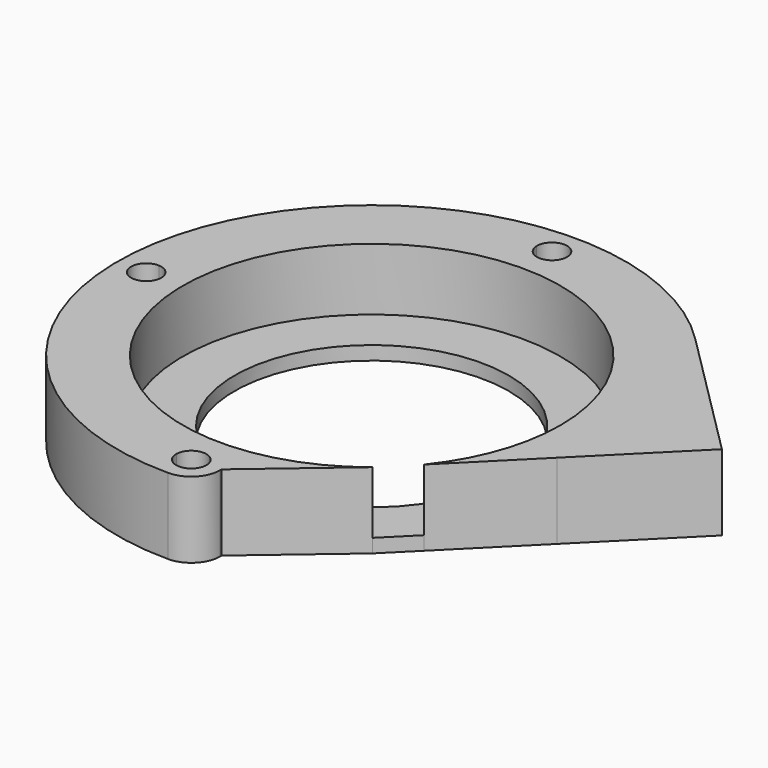
from build123d import *

# Parameters (mm, degrees)
F0_R     = 15
F1_DEPTH = 1.5
F2_DEPTH = 6.8


with BuildPart() as f1:
    # F0 (on Top) → F1 (new body)
    with BuildSketch(Plane.XY):
        with BuildLine():
            ThreePointArc((24.1652138662, -4.8646622494), (24.5285040494, -2.4443790825), (24.65, 0))
            ThreePointArc((24.65, 0), (18.0037803541, 16.8370541652), (1.6490756219, 24.5947768763))
            ThreePointArc((1.6490756219, 24.5947768763), (0, 23), (-1.6490756219, 24.5947768763))
            ThreePointArc((-1.6490756219, 24.5947768763), (-17.4301821562, 17.4301821562), (-24.5947768763, 1.6490756219))
            ThreePointArc((-24.5947768763, 1.6490756219), (-23.4639101733, 1.1470357113), (-23, 0))
            ThreePointArc((-23, 0), (-23.4639101733, -1.1470357113), (-24.5947768763, -1.6490756219))
            ThreePointArc((-24.5947768763, -1.6490756219), (-17.9529932576, -16.8911969112), (-3.1435634706, -24.4487322515))
            ThreePointArc((-3.1435634706, -24.4487322515), (0, -21.5), (3.1435634706, -24.4487322515))
            Line((3.1435634706, -24.4487322515), (12.969203616, -16.0692954907))
            ThreePointArc((12.969203616, -16.0692954907), (-18.6311104697, 8.9052918349), (20.65, 0))
            ThreePointArc((20.65, 0), (19.4738226895, -6.8696964896), (16.0792755585, -12.9568282197))
            Line((16.0792755585, -12.9568282197), (24.1652138662, -4.8646622494))
        make_face()
        with BuildLine():
            ThreePointArc((1.6490756219, 24.5947768763), (18.0037803541, 16.8370541652), (24.65, 0))
            ThreePointArc((24.65, 0), (24.5285040494, -2.4443790825), (24.1652138662, -4.8646622494))
            Line((24.1652138662, -4.8646622494), (27.771636901, -1.2554616043))
            ThreePointArc((27.771636901, -1.2554616043), (27.7929083207, -0.6278909749), (27.8, 0))
            ThreePointArc((27.8, 0), (25.6818028962, 10.6435426433), (19.65, 19.6651341211))
            ThreePointArc((19.65, 19.6651341211), (-25.6858981613, 10.6336557988), (7.1e-09, -27.8))
            ThreePointArc((7.1e-09, -27.8), (-2.2974435124, -26.8050529709), (-3.1435634706, -24.4487322515))
            ThreePointArc((-3.1435634706, -24.4487322515), (-17.9529932576, -16.8911969112), (-24.5947768763, -1.6490756219))
            ThreePointArc((-24.5947768763, -1.6490756219), (-26.3, 0), (-24.5947768763, 1.6490756219))
            ThreePointArc((-24.5947768763, 1.6490756219), (-17.4301821562, 17.4301821562), (-1.6490756219, 24.5947768763))
            ThreePointArc((-1.6490756219, 24.5947768763), (-0.0276154299, 26.2997688893), (1.65, 24.65))
            ThreePointArc((1.65, 24.65), (1.6497688893, 24.6223845701), (1.6490756219, 24.5947768763))
        make_face()
        with BuildLine():
            ThreePointArc((3.15, -24.65), (3.1483904564, -24.549314679), (3.1435634706, -24.4487322515))
            ThreePointArc((3.1435634706, -24.4487322515), (2.3974318813, -24.5331371898), (1.6490756219, -24.5947768763))
            ThreePointArc((1.6490756219, -24.5947768763), (1.6497688893, -24.6223845701), (1.65, -24.65))
            ThreePointArc((1.65, -24.65), (-0.0276154299, -26.2997688893), (-1.6490756219, -24.5947768763))
            ThreePointArc((-1.6490756219, -24.5947768763), (-2.3974318813, -24.5331371898), (-3.1435634706, -24.4487322515))
            ThreePointArc((-3.1435634706, -24.4487322515), (-2.2974435124, -26.8050529709), (7.1e-09, -27.8))
            ThreePointArc((7.1e-09, -27.8), (2.2273863633, -26.8773863582), (3.15, -24.65))
        make_face()
        with BuildLine():
            ThreePointArc((1.6490756219, -24.5947768763), (2.3974318813, -24.5331371898), (3.1435634706, -24.4487322515))
            ThreePointArc((3.1435634706, -24.4487322515), (0, -21.5), (-3.1435634706, -24.4487322515))
            ThreePointArc((-3.1435634706, -24.4487322515), (-2.3974318813, -24.5331371898), (-1.6490756219, -24.5947768763))
            ThreePointArc((-1.6490756219, -24.5947768763), (0, -23), (1.6490756219, -24.5947768763))
        make_face()
        with BuildLine():
            Line((12.969203616, -16.0692954907), (16.0792755585, -12.9568282197))
            ThreePointArc((16.0792755585, -12.9568282197), (19.4738226895, -6.8696964896), (20.65, 0))
            ThreePointArc((20.65, 0), (-18.6311104697, 8.9052918349), (12.969203616, -16.0692954907))
        make_face()
        Circle(F0_R, mode=Mode.SUBTRACT)
        with BuildLine():
            ThreePointArc((27.8, 0), (27.7929083207, -0.6278909749), (27.771636901, -1.2554616043))
            Line((27.771636901, -1.2554616043), (34.1742395873, 5.1520722659))
            Line((34.1742395873, 5.1520722659), (19.65, 19.6651341211))
            ThreePointArc((19.65, 19.6651341211), (25.6818028962, 10.6435426433), (27.8, 0))
        make_face()
    extrude(amount=-F1_DEPTH)

    # F0 (on Top) → F2 (join)
    with BuildSketch(Plane.XY):
        with BuildLine():
            ThreePointArc((24.1652138662, -4.8646622494), (24.5285040494, -2.4443790825), (24.65, 0))
            ThreePointArc((24.65, 0), (18.0037803541, 16.8370541652), (1.6490756219, 24.5947768763))
            ThreePointArc((1.6490756219, 24.5947768763), (0, 23), (-1.6490756219, 24.5947768763))
            ThreePointArc((-1.6490756219, 24.5947768763), (-17.4301821562, 17.4301821562), (-24.5947768763, 1.6490756219))
            ThreePointArc((-24.5947768763, 1.6490756219), (-23.4639101733, 1.1470357113), (-23, 0))
            ThreePointArc((-23, 0), (-23.4639101733, -1.1470357113), (-24.5947768763, -1.6490756219))
            ThreePointArc((-24.5947768763, -1.6490756219), (-17.9529932576, -16.8911969112), (-3.1435634706, -24.4487322515))
            ThreePointArc((-3.1435634706, -24.4487322515), (0, -21.5), (3.1435634706, -24.4487322515))
            Line((3.1435634706, -24.4487322515), (12.969203616, -16.0692954907))
            ThreePointArc((12.969203616, -16.0692954907), (-18.6311104697, 8.9052918349), (20.65, 0))
            ThreePointArc((20.65, 0), (19.4738226895, -6.8696964896), (16.0792755585, -12.9568282197))
            Line((16.0792755585, -12.9568282197), (24.1652138662, -4.8646622494))
        make_face()
        with BuildLine():
            ThreePointArc((1.6490756219, 24.5947768763), (18.0037803541, 16.8370541652), (24.65, 0))
            ThreePointArc((24.65, 0), (24.5285040494, -2.4443790825), (24.1652138662, -4.8646622494))
            Line((24.1652138662, -4.8646622494), (27.771636901, -1.2554616043))
            ThreePointArc((27.771636901, -1.2554616043), (27.7929083207, -0.6278909749), (27.8, 0))
            ThreePointArc((27.8, 0), (25.6818028962, 10.6435426433), (19.65, 19.6651341211))
            ThreePointArc((19.65, 19.6651341211), (-25.6858981613, 10.6336557988), (7.1e-09, -27.8))
            ThreePointArc((7.1e-09, -27.8), (-2.2974435124, -26.8050529709), (-3.1435634706, -24.4487322515))
            ThreePointArc((-3.1435634706, -24.4487322515), (-17.9529932576, -16.8911969112), (-24.5947768763, -1.6490756219))
            ThreePointArc((-24.5947768763, -1.6490756219), (-26.3, 0), (-24.5947768763, 1.6490756219))
            ThreePointArc((-24.5947768763, 1.6490756219), (-17.4301821562, 17.4301821562), (-1.6490756219, 24.5947768763))
            ThreePointArc((-1.6490756219, 24.5947768763), (-0.0276154299, 26.2997688893), (1.65, 24.65))
            ThreePointArc((1.65, 24.65), (1.6497688893, 24.6223845701), (1.6490756219, 24.5947768763))
        make_face()
        with BuildLine():
            ThreePointArc((3.15, -24.65), (3.1483904564, -24.549314679), (3.1435634706, -24.4487322515))
            ThreePointArc((3.1435634706, -24.4487322515), (2.3974318813, -24.5331371898), (1.6490756219, -24.5947768763))
            ThreePointArc((1.6490756219, -24.5947768763), (1.6497688893, -24.6223845701), (1.65, -24.65))
            ThreePointArc((1.65, -24.65), (-0.0276154299, -26.2997688893), (-1.6490756219, -24.5947768763))
            ThreePointArc((-1.6490756219, -24.5947768763), (-2.3974318813, -24.5331371898), (-3.1435634706, -24.4487322515))
            ThreePointArc((-3.1435634706, -24.4487322515), (-2.2974435124, -26.8050529709), (7.1e-09, -27.8))
            ThreePointArc((7.1e-09, -27.8), (2.2273863633, -26.8773863582), (3.15, -24.65))
        make_face()
        with BuildLine():
            ThreePointArc((1.6490756219, -24.5947768763), (2.3974318813, -24.5331371898), (3.1435634706, -24.4487322515))
            ThreePointArc((3.1435634706, -24.4487322515), (0, -21.5), (-3.1435634706, -24.4487322515))
            ThreePointArc((-3.1435634706, -24.4487322515), (-2.3974318813, -24.5331371898), (-1.6490756219, -24.5947768763))
            ThreePointArc((-1.6490756219, -24.5947768763), (0, -23), (1.6490756219, -24.5947768763))
        make_face()
        with BuildLine():
            ThreePointArc((27.8, 0), (27.7929083207, -0.6278909749), (27.771636901, -1.2554616043))
            Line((27.771636901, -1.2554616043), (34.1742395873, 5.1520722659))
            Line((34.1742395873, 5.1520722659), (19.65, 19.6651341211))
            ThreePointArc((19.65, 19.6651341211), (25.6818028962, 10.6435426433), (27.8, 0))
        make_face()
    extrude(amount=F2_DEPTH)


solid = f1.part
